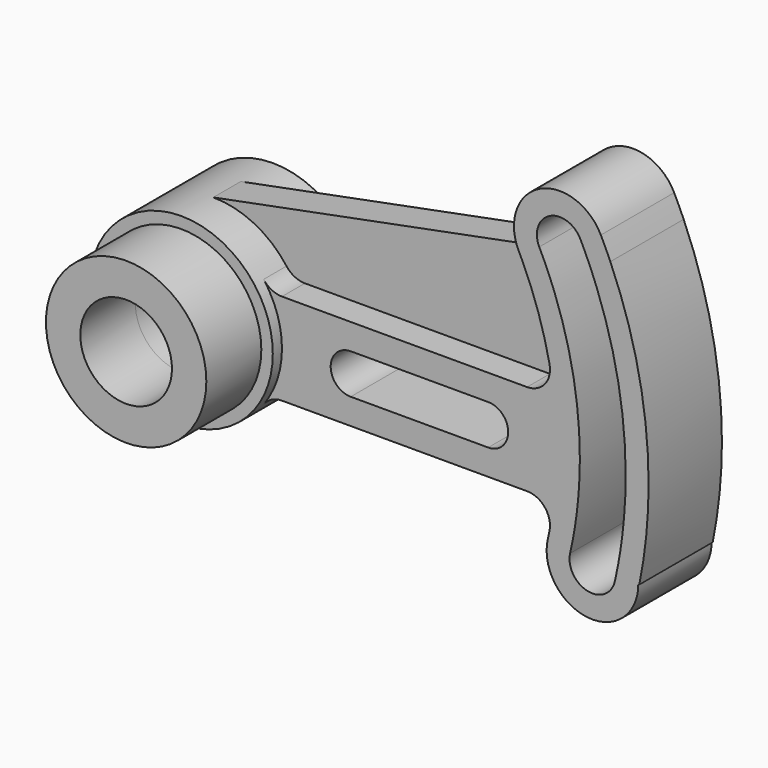
from build123d import *

# Parameters (mm, degrees)
F0_W         = 38.1
F0_H         = 7.1501
F0_R         = 22.225
F0_R_2       = 12.7
F1_DEPTH     = 12.7
F2_DEPTH     = 15.875
F3_DEPTH     = 4.7625
F5_DEPTH     = 34.925
F6_T1_DEPTH  = 9.525
F6_T3_DEPTH  = 25.4
F6_T5_DEPTH  = 16.4448868597
F6_T7_DEPTH  = 16.4448868597
F6_T12_DEPTH = 27.2444917505
F6_T17_DEPTH = 27.2444917505


# Not quite as in the source:
# - a fillet or chamfer that OpenCascade refuses, or shapes differently, is made with other operations: its cross-section is extruded or revolved along the edge and cut away or added


with BuildPart() as f1:
    # F0 (on Front) → F1 (new body)
    with BuildSketch(Plane.XZ):
        with BuildLine():
            ThreePointArc((113.7674148927, 56.4444444444), (96.7462289589, 62.1767414893), (91.0139319141, 45.1555555556))
            ThreePointArc((91.0139319141, 45.1555555556), (95.1042946992, 40.3981402923), (100.9729543694, 38.1793790668))
            ThreePointArc((100.9729543694, 38.1793790668), (98.95897617, 43.1314680412), (96.7023026588, 47.9777777778))
            ThreePointArc((96.7023026588, 47.9777777778), (99.5684511812, 56.4883707446), (108.079044148, 53.6222222222))
            ThreePointArc((108.079044148, 53.6222222222), (108.7656354529, 52.2155057864), (109.4339184165, 50.8))
            Line((109.4339184165, 50.8), (115.0906734034, 50.8))
            ThreePointArc((115.0906734034, 50.8), (114.7554341555, 53.6987396474), (113.7674148927, 56.4444444444))
        make_face()
        with BuildLine():
            ThreePointArc((91.0139319141, 45.1555555556), (91.4748276489, 44.2144309769), (91.9259920573, 43.2686027539))
            ThreePointArc((91.9259920573, 43.2686027539), (97.5691447351, 28.3341136382), (100.8031249516, 12.7))
            ThreePointArc((100.8031249516, 12.7), (101.4005855384, 6.3624879144), (101.6, 0))
            Line((101.6, 0), (107.95, 0))
            ThreePointArc((107.95, 0), (106.1914142579, 19.405824845), (100.9729543694, 38.1793790668))
            ThreePointArc((100.9729543694, 38.1793790668), (95.1042946992, 40.3981402923), (91.0139319141, 45.1555555556))
        make_face()
        with BuildLine():
            ThreePointArc((101.6, 0), (101.4005855384, -6.3624879144), (100.8031249516, -12.7))
            ThreePointArc((100.8031249516, -12.7), (100.0533339134, -17.6604182514), (99.0595979732, -22.5777777778))
            ThreePointArc((99.0595979732, -22.5777777778), (101.9216501545, -16.9945237972), (107.1072287434, -13.462691072))
            ThreePointArc((107.1072287434, -13.462691072), (107.7391011724, -6.744522116), (107.95, 0))
            Line((107.95, 0), (101.6, 0))
        make_face()
        with BuildLine():
            ThreePointArc((124.4340789334, -25.4), (126.3568914317, -12.7646381747), (127, 0))
            Line((127, 0), (120.65, 0))
            ThreePointArc((120.65, 0), (120.3936458808, -7.8608225729), (119.625672913, -15.6882401853))
            ThreePointArc((119.625672913, -15.6882401853), (122.957733543, -20.0447240945), (124.1420477199, -25.4))
            Line((124.1420477199, -25.4), (124.4340789334, -25.4))
        make_face()
        with BuildLine():
            Line((116.3974226519, 50.8), (115.0906734034, 50.8))
            ThreePointArc((115.0906734034, 50.8), (114.4576498997, 46.8404446919), (112.6216847044, 43.2756124663))
            ThreePointArc((112.6216847044, 43.2756124663), (118.6259431145, 22.0070016178), (120.65, 0))
            Line((120.65, 0), (127, 0))
            ThreePointArc((127, 0), (124.3211017422, 25.9473247485), (116.3974226519, 50.8))
        make_face()
        with BuildLine():
            Line((117.9460151934, -25.4), (124.1420477199, -25.4))
            ThreePointArc((124.1420477199, -25.4), (122.957733543, -20.0447240945), (119.625672913, -15.6882401853))
            ThreePointArc((119.625672913, -15.6882401853), (118.885055062, -20.5612787271), (117.9460151934, -25.4))
        make_face()
        with BuildLine():
            ThreePointArc((107.1072287434, -13.462691072), (101.9216501545, -16.9945237972), (99.0595979732, -22.5777777778))
            ThreePointArc((99.0595979732, -22.5777777778), (108.6198254977, -37.7824497467), (123.8244974665, -28.2222222222))
            ThreePointArc((123.8244974665, -28.2222222222), (124.0624104679, -26.8200155312), (124.1420477199, -25.4))
            Line((124.1420477199, -25.4), (117.9460151934, -25.4))
            ThreePointArc((117.9460151934, -25.4), (117.791757, -26.1060238805), (117.6332725932, -26.8111111111))
            ThreePointArc((117.6332725932, -26.8111111111), (110.0309366088, -31.5912248733), (105.2508228466, -23.9888888889))
            ThreePointArc((105.2508228466, -23.9888888889), (106.3093868334, -18.7487805232), (107.1072287434, -13.462691072))
        make_face()
        with BuildLine():
            ThreePointArc((112.6216847044, 43.2756124663), (114.4576498997, 46.8404446919), (115.0906734034, 50.8))
            Line((115.0906734034, 50.8), (109.4339184165, 50.8))
            ThreePointArc((109.4339184165, 50.8), (111.091524525, 47.064802971), (112.6216847044, 43.2756124663))
        make_face()
        with BuildLine():
            ThreePointArc((116.3974226519, 50.8), (115.1170189362, 53.6383440391), (113.7674148927, 56.4444444444))
            ThreePointArc((113.7674148927, 56.4444444444), (114.7554341555, 53.6987396474), (115.0906734034, 50.8))
            Line((115.0906734034, 50.8), (116.3974226519, 50.8))
        make_face()
        with BuildLine():
            ThreePointArc((21.9970452561, 12.7), (24.5345159877, 6.5740037456), (25.4, 0))
            Line((25.4, 0), (38.9001, 0))
            ThreePointArc((38.9001, 0), (40.5256280751, 3.9243719249), (44.45, 5.5499))
            Line((44.45, 5.5499), (44.45, 12.7))
            Line((44.45, 12.7), (21.9970452561, 12.7))
        make_face()
        with Locations((63.5, 9.12495)):
            Rectangle(F0_W, F0_H)
        with BuildLine():
            Line((82.55, 12.7), (82.55, 5.5499))
            ThreePointArc((82.55, 5.5499), (86.4743719249, 3.9243719249), (88.0999, 0))
            Line((88.0999, 0), (101.6, 0))
            ThreePointArc((101.6, 0), (101.4005855384, 6.3624879144), (100.8031249516, 12.7))
            Line((100.8031249516, 12.7), (82.55, 12.7))
        make_face()
        with BuildLine():
            ThreePointArc((88.0999, 0), (86.4743719249, -3.9243719249), (82.55, -5.5499))
            Line((82.55, -5.5499), (82.55, -12.7))
            Line((82.55, -12.7), (100.8031249516, -12.7))
            ThreePointArc((100.8031249516, -12.7), (101.4005855384, -6.3624879144), (101.6, 0))
            Line((101.6, 0), (88.0999, 0))
        make_face()
        with Locations((63.5, -9.12495)):
            Rectangle(F0_W, F0_H)
        with BuildLine():
            Line((38.9001, 0), (25.4, 0))
            ThreePointArc((25.4, 0), (24.5345159877, -6.5740037456), (21.9970452561, -12.7))
            Line((21.9970452561, -12.7), (44.45, -12.7))
            Line((44.45, -12.7), (44.45, -5.5499))
            ThreePointArc((44.45, -5.5499), (40.5256280751, -3.9243719249), (38.9001, 0))
        make_face()
        with BuildLine():
            ThreePointArc((21.9970452561, -12.7), (24.5345159877, -6.5740037456), (25.4, 0))
            ThreePointArc((25.4, 0), (24.5345159877, 6.5740037456), (21.9970452561, 12.7))
            ThreePointArc((21.9970452561, 12.7), (12.7, 21.9970452561), (0, 25.4))
            ThreePointArc((0, 25.4), (-21.9970452561, -12.7), (21.9970452561, -12.7))
        make_face()
        Circle(F0_R, mode=Mode.SUBTRACT)
        Circle(F0_R)
        Circle(F0_R_2, mode=Mode.SUBTRACT)
    extrude(amount=F1_DEPTH)

    # F0 (on Front) → F2 (join)
    with BuildSketch(Plane.XZ):
        with BuildLine():
            ThreePointArc((21.9970452561, -12.7), (24.5345159877, -6.5740037456), (25.4, 0))
            ThreePointArc((25.4, 0), (24.5345159877, 6.5740037456), (21.9970452561, 12.7))
            ThreePointArc((21.9970452561, 12.7), (12.7, 21.9970452561), (0, 25.4))
            ThreePointArc((0, 25.4), (-21.9970452561, -12.7), (21.9970452561, -12.7))
        make_face()
        Circle(F0_R, mode=Mode.SUBTRACT)
        Circle(F0_R)
        Circle(F0_R_2, mode=Mode.SUBTRACT)
    extrude(amount=F2_DEPTH)

    # F0 (on Front) → F3 (join)
    with BuildSketch(Plane.XZ):
        with BuildLine():
            ThreePointArc((0, 25.4), (12.7, 21.9970452561), (21.9970452561, 12.7))
            Line((21.9970452561, 12.7), (44.45, 12.7))
            Line((44.45, 12.7), (82.55, 12.7))
            Line((82.55, 12.7), (100.8031249516, 12.7))
            ThreePointArc((100.8031249516, 12.7), (97.5691447351, 28.3341136382), (91.9259920573, 43.2686027539))
            Line((91.9259920573, 43.2686027539), (0, 25.4))
        make_face()
    extrude(amount=F3_DEPTH)

    # F4: F1 across face


with BuildPart() as f1_1:
    add(f1.part)
    add(f1.part.mirror(Plane.XZ))

    # F0 (on Front) → F5 (join)
    with BuildSketch(Plane.XZ):
        Circle(F0_R)
        Circle(F0_R_2, mode=Mode.SUBTRACT)
    extrude(amount=F5_DEPTH)

    # F6: fillet of radius 6.35 on 7 edges, made by hand

    # F6_s2 → F6_t1 (join)
    with BuildSketch(Plane.XZ.offset(-4.7625)):
        with BuildLine():
            ThreePointArc((84.7437823747, 41.8725226155), (88.7059686824, 44.4242725365), (89.8183213038, 49.0039034869))
            Line((89.8183213038, 49.0039034869), (90.4469389088, 49.0937083126))
            ThreePointArc((90.4469389088, 49.0937083126), (91.5827689886, 45.4377777778), (92.5005295077, 43.5390315211))
            Line((92.5005295077, 43.5390315211), (92.0471557694, 42.6452694924))
            Line((92.0471557694, 42.6452694924), (84.8649460867, 41.249189354))
            Line((84.8649460867, 41.249189354), (84.7437823747, 41.8725226155))
        make_face()
    extrude(amount=F6_T1_DEPTH)

    # F6_s4 → F6_t3 (join)
    with BuildSketch(Plane.XZ.offset(-12.7)):
        with BuildLine():
            ThreePointArc((93.3255592, -12.7), (98.2442480497, -15.0339073716), (99.5472631467, -20.32))
            ThreePointArc((99.5472631467, -20.32), (100.247621432, -16.5219368483), (100.8031249516, -12.7))
            Line((100.8031249516, -12.7), (93.3255592, -12.7))
        make_face()
        with BuildLine():
            ThreePointArc((20.32, -15.24), (22.5601936686, -13.3703873372), (25.4, -12.7))
            Line((25.4, -12.7), (21.9970452561, -12.7))
            ThreePointArc((21.9970452561, -12.7), (21.1966030251, -13.9951427359), (20.32, -15.24))
        make_face()
    extrude(amount=F6_T3_DEPTH)

    # F6_s6 → F6_t5 (join)
    with BuildSketch(Plane.XZ.offset(-3.7448868597)):
        with BuildLine():
            ThreePointArc((25.4, 12.7), (22.5601936686, 13.3703873372), (20.32, 15.24))
            ThreePointArc((20.32, 15.24), (21.1966030251, 13.9951427359), (21.9970452561, 12.7))
            Line((21.9970452561, 12.7), (25.4, 12.7))
        make_face()
    extrude(amount=F6_T5_DEPTH)

    # F6_s8 → F6_t7 (join)
    with BuildSketch(Plane.XZ.offset(-12.7)):
        with BuildLine():
            ThreePointArc((25.4, 12.7), (22.5601936686, 13.3703873372), (20.32, 15.24))
            ThreePointArc((20.32, 15.24), (21.1966030251, 13.9951427359), (21.9970452561, 12.7))
            Line((21.9970452561, 12.7), (25.4, 12.7))
        make_face()
    extrude(amount=F6_T7_DEPTH)


with BuildPart() as f6_tool10:
    # F6_s11 → F6_t12 (new body)
    with BuildSketch(Plane.XZ.offset(-14.5444917505)):
        with BuildLine():
            ThreePointArc((93.3255592, 12.7), (98.2442480497, 15.0339073716), (99.5472631467, 20.32))
            ThreePointArc((99.5472631467, 20.32), (100.247621432, 16.5219368483), (100.8031249516, 12.7))
            Line((100.8031249516, 12.7), (93.3255592, 12.7))
        make_face()
    extrude(amount=F6_T12_DEPTH)

    split(bisect_by=Plane.XZ.offset(-12.7), keep=Keep.TOP)


with BuildPart() as f1_2:
    add(f1_1.part)

    # F6_t9: union F6_tool10
    add(f6_tool10.part)


with BuildPart() as f6_tool15:
    # F6_s16 → F6_t17 (new body)
    with BuildSketch(Plane.XZ.offset(14.5444917505)):
        with BuildLine():
            ThreePointArc((93.3255592, 12.7), (98.2442480497, 15.0339073716), (99.5472631467, 20.32))
            ThreePointArc((99.5472631467, 20.32), (100.247621432, 16.5219368483), (100.8031249516, 12.7))
            Line((100.8031249516, 12.7), (93.3255592, 12.7))
        make_face()
    extrude(amount=-F6_T17_DEPTH)

    split(bisect_by=Plane.XZ.offset(12.7), keep=Keep.BOTTOM)


with BuildPart() as f1_3:
    add(f1_2.part)

    # F6_t14: union F6_tool15
    add(f6_tool15.part)


solid = f1_3.part
